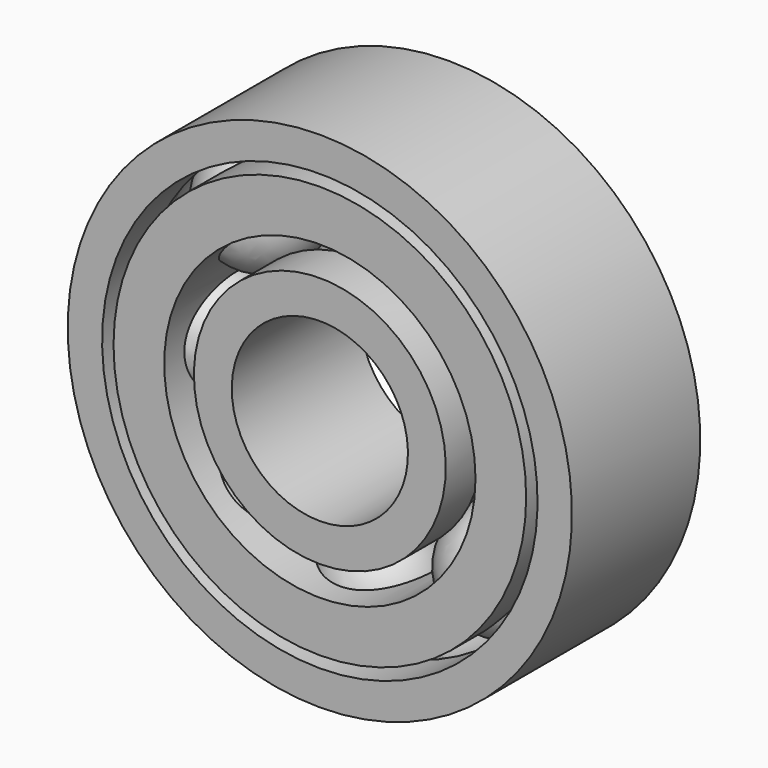
from build123d import *

# Parameters (mm, degrees)
F7_COUNT = 8
F8_R     = 8.9924805532
F8_R_2   = 6.7840576958
F9_DEPTH = 6.99


with BuildPart() as f4:
    # F2 (on Right) → F4 (revolve)
    with BuildSketch(Plane.YZ):
        with BuildLine():
            Line((0, -9.99), (0, -4.99))
            ThreePointArc((0, -4.99), (-2.5, -7.49), (0, -9.99))
        make_face()
    revolve(axis=Axis((0, 0, -7.49), (0, 0, 1)))


with BuildPart() as f6:
    # F1 (on Right) → F6 (revolve)
    with BuildSketch(Plane.YZ):
        with BuildLine():
            ThreePointArc((1.5, -9.49), (0.790569415, -9.8617082451), (0, -9.99))
            Line((0, -9.99), (0, -10.99))
            Line((0, -10.99), (3.495, -10.99))
            Line((3.495, -10.99), (3.495, -9.49))
            Line((3.495, -9.49), (1.5, -9.49))
        make_face()
        with BuildLine():
            ThreePointArc((0, -9.99), (-0.790569415, -9.8617082451), (-1.5, -9.49))
            Line((-1.5, -9.49), (-3.495, -9.49))
            Line((-3.495, -9.49), (-3.495, -10.99))
            Line((-3.495, -10.99), (0, -10.99))
            Line((0, -10.99), (0, -9.99))
        make_face()
    revolve(axis=Axis((0, -0.1336969435, 0), (0, 1, 0)))


with BuildPart() as f6b:
    # F3 (on Right) → F6, piece 2 (revolve)
    with BuildSketch(Plane.YZ):
        with BuildLine():
            Line((-3.495, -5.49), (-1.5, -5.49))
            ThreePointArc((-1.5, -5.49), (-0.790569415, -5.1182917549), (0, -4.99))
            ThreePointArc((0, -4.99), (0.790569415, -5.1182917549), (1.5, -5.49))
            Line((1.5, -5.49), (3.495, -5.49))
            Line((3.495, -5.49), (3.495, -3.84))
            Line((3.495, -3.84), (0, -3.84))
            Line((0, -3.84), (-3.495, -3.84))
            Line((-3.495, -3.84), (-3.495, -5.49))
        make_face()
    revolve(axis=Axis((0, -0.1336969435, 0), (0, 1, 0)))


with BuildPart() as f7_1:
    # F7: instance of F4
    add(f4.part.rotate(Axis((0, -0.1336969435, 0), (0, 1, 0)), 1 * 360 / F7_COUNT))


with BuildPart() as f7_2:
    # F7: instance of F4
    add(f4.part.rotate(Axis((0, -0.1336969435, 0), (0, 1, 0)), 2 * 360 / F7_COUNT))


with BuildPart() as f7_3:
    # F7: instance of F4
    add(f4.part.rotate(Axis((0, -0.1336969435, 0), (0, 1, 0)), 3 * 360 / F7_COUNT))


with BuildPart() as f7_4:
    # F7: instance of F4
    add(f4.part.rotate(Axis((0, -0.1336969435, 0), (0, 1, 0)), 4 * 360 / F7_COUNT))


with BuildPart() as f7_5:
    # F7: instance of F4
    add(f4.part.rotate(Axis((0, -0.1336969435, 0), (0, 1, 0)), 5 * 360 / F7_COUNT))


with BuildPart() as f7_6:
    # F7: instance of F4
    add(f4.part.rotate(Axis((0, -0.1336969435, 0), (0, 1, 0)), 6 * 360 / F7_COUNT))


with BuildPart() as f7_7:
    # F7: instance of F4
    add(f4.part.rotate(Axis((0, -0.1336969435, 0), (0, 1, 0)), 7 * 360 / F7_COUNT))


with BuildPart() as f9:
    # F8 (on face) → F9 (new body)
    with BuildSketch(Plane.XZ.offset(3.495)):
        Circle(F8_R)
        Circle(F8_R_2, mode=Mode.SUBTRACT)
    extrude(amount=-F9_DEPTH)

    # F10: cut F7_7, F7_6, F7_5, F7_4, F7_3, F7_2, F7_1, F4
    add(f7_7.part, mode=Mode.SUBTRACT)
    add(f7_6.part, mode=Mode.SUBTRACT)
    add(f7_5.part, mode=Mode.SUBTRACT)
    add(f7_4.part, mode=Mode.SUBTRACT)
    add(f7_3.part, mode=Mode.SUBTRACT)
    add(f7_2.part, mode=Mode.SUBTRACT)
    add(f7_1.part, mode=Mode.SUBTRACT)
    add(f4.part, mode=Mode.SUBTRACT)


solid = Compound([f4.part, f6.part, f6b.part, f7_1.part, f7_2.part, f7_3.part, f7_4.part, f7_5.part, f7_6.part, f7_7.part, f9.part])
